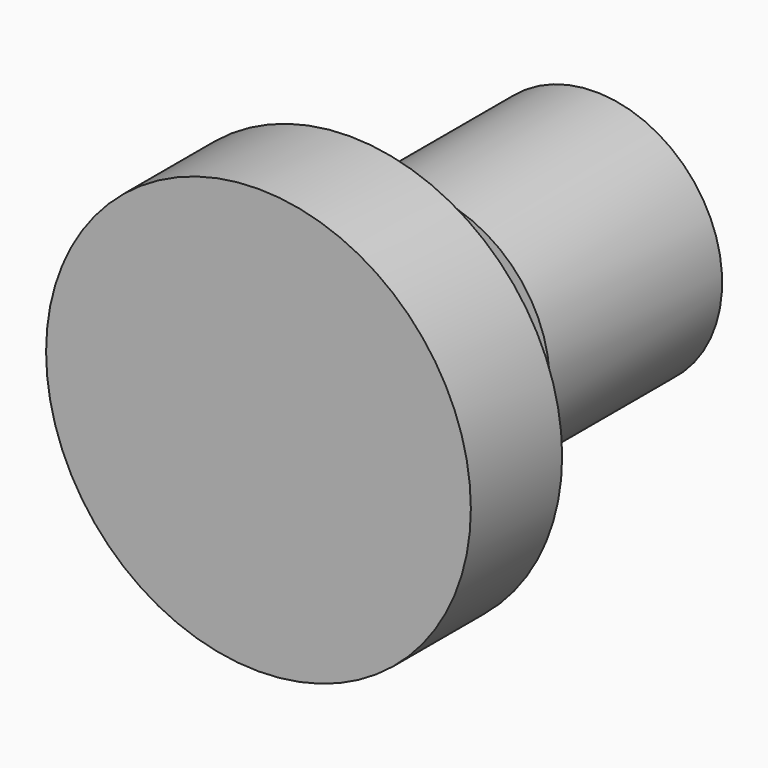
from build123d import *

# Parameters (mm, degrees)
F4_R     = 11.5
F5_DEPTH = 8


# Not quite as in the source:
# - a feature names something its author has since deleted; it is built from what else it names


with BuildPart() as f1:
    # F0 (on Top) → F1 (revolve)
    with BuildSketch(Plane.XY):
        Polygon((0, 20), (0, 0), (16.75, 0), (16.75, 9), (11.75, 9), (11.75, 1), (3.9, 1), (3.9, 20), align=None)
    revolve(axis=Axis((0, 10, 0), (0, 1, 0)))

    # F4 (on Front) → F5 (join)
    with BuildSketch(Plane.XZ):
        Circle(F4_R)
    extrude(amount=-F5_DEPTH)


with BuildPart() as f3:
    # F2 (on Top) → F3 (revolve)
    with BuildSketch(Plane.XY):
        Polygon((-10, 16.2120937904), (-4, 16.2120937904), (-4, 28.2120937904), (0, 28.2120937904), (0, 33.2120937904), (-10, 33.2120937904), align=None)
    revolve(axis=Axis((0, 30.7120937904, 0), (0, 1, 0)))


solid = Compound([f1.part, f3.part])
